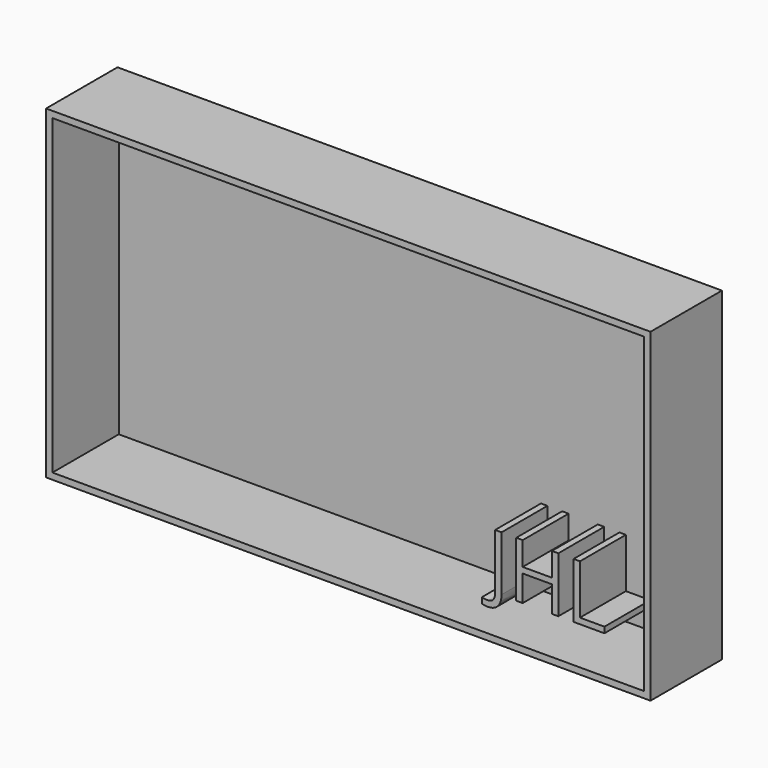
from build123d import *

# Parameters (mm, degrees)
F0_W         = 237.0375022292
F0_H         = 127.3781321943
F0_R         = 8.3758696303
F0_TEXT_SIZE = 30.4503935493
F1_DEPTH     = 35
F2_T         = -2.5
F3_DEPTH     = 25
F4_DEPTH     = 50


# Not quite as in the source:
# - Text() gives the source's letters only with a copy of the font that has no kerning and outlines rounded to 1/6400 em; it was checked with that copy


with BuildPart() as f1:
    # F0 (on Front) → F1 (new body)
    with BuildSketch(Plane.XZ):
        with Locations((-2.460937947, -3.9374995977)):
            Rectangle(F0_W, F0_H)
        with BuildLine():
            add(Edge.make_bspline(
                [(48.2012823656, -61.0663670616), (46.773920168, -62.61981292), (44.0952371104, -62.61981292)],
                knots=[0, 0, 0, 1, 1, 1], degree=2))
            add(Edge.make_bspline(
                [(44.0952371104, -62.61981292), (42.7011800307, -62.61981292), (41.8970993261, -62.2201515046)],
                knots=[0, 0, 0, 1, 1, 1], degree=2))
            Line((41.8970993261, -62.2201515046), (41.8970993261, -60.0648345862))
            add(Edge.make_bspline(
                [(41.8970993261, -60.0648345862), (42.9533473523, -60.3598227737), (44.0952371104, -60.3598227737)],
                knots=[0, 0, 0, 1, 1, 1], degree=2))
            add(Edge.make_bspline(
                [(44.0952371104, -60.3598227737), (45.570178048, -60.3598227737), (46.3361957607, -59.4677214002)],
                knots=[0, 0, 0, 1, 1, 1], degree=2))
            add(Edge.make_bspline(
                [(46.3361957607, -59.4677214002), (47.1022134734, -58.5756200267), (47.1022134734, -56.8960905075)],
                knots=[0, 0, 0, 1, 1, 1], degree=2))
            Line((47.1022134734, -56.8960905075), (47.1022134734, -35.1573642377))
            Line((47.1022134734, -35.1573642377), (49.6286445632, -35.1573642377))
            Line((49.6286445632, -35.1573642377), (49.6286445632, -56.6867440519))
            add(Edge.make_bspline(
                [(49.6286445632, -56.6867440519), (49.6286445632, -59.5129212031), (48.2012823656, -61.0663670616)],
                knots=[0, 0, 0, 1, 1, 1], degree=2))
        make_face(mode=Mode.SUBTRACT)
        Polygon((71.9002527201, -35.1573642377), (71.9002527201, -56.8960905075), (69.3738216303, -56.8960905075), (69.3738216303, -46.6666614245), (57.9216189314, -46.6666614245), (57.9216189314, -56.8960905075), (55.3951878416, -56.8960905075), (55.3951878416, -35.1573642377), (57.9216189314, -35.1573642377), (57.9216189314, -44.4066712783), (69.3738216303, -44.4066712783), (69.3738216303, -35.1573642377), align=None, mode=Mode.SUBTRACT)
        Polygon((89.98017389, -56.8960905075), (77.8618688322, -56.8960905075), (77.8618688322, -35.1573642377), (80.388299922, -35.1573642377), (80.388299922, -54.6075531173), (89.98017389, -54.6075531173), align=None, mode=Mode.SUBTRACT)
        with Locations((0, 16.6359394789)):
            Circle(F0_R, mode=Mode.SUBTRACT)
        with Locations((0, 16.6359394789)):
            Circle(F0_R)
        with Locations((44.2760363221, -56.8960905075)):
            Text('JHL', F0_TEXT_SIZE, font='Open Sans', text_align=(TextAlign.LEFT, TextAlign.BOTTOM))
    extrude(amount=F1_DEPTH)

    # F2
    f2_openings = [f1.faces().sort_by_distance(p)[0] for p in [
        (-2.460938, -35, -3.9375),
    ]]
    offset(amount=F2_T, openings=f2_openings)

    # F0 (on Front) → F3 (join)
    with BuildSketch(Plane.XZ):
        with Locations((44.2760363221, -56.8960905075)):
            Text('JHL', F0_TEXT_SIZE, font='Open Sans', text_align=(TextAlign.LEFT, TextAlign.BOTTOM))
    extrude(amount=F3_DEPTH)

    # F0 (on Front) → F4 (join)
    with BuildSketch(Plane.XZ):
        with Locations((0, 16.6359394789)):
            Circle(F0_R)
    extrude(amount=-F4_DEPTH)


solid = f1.part
